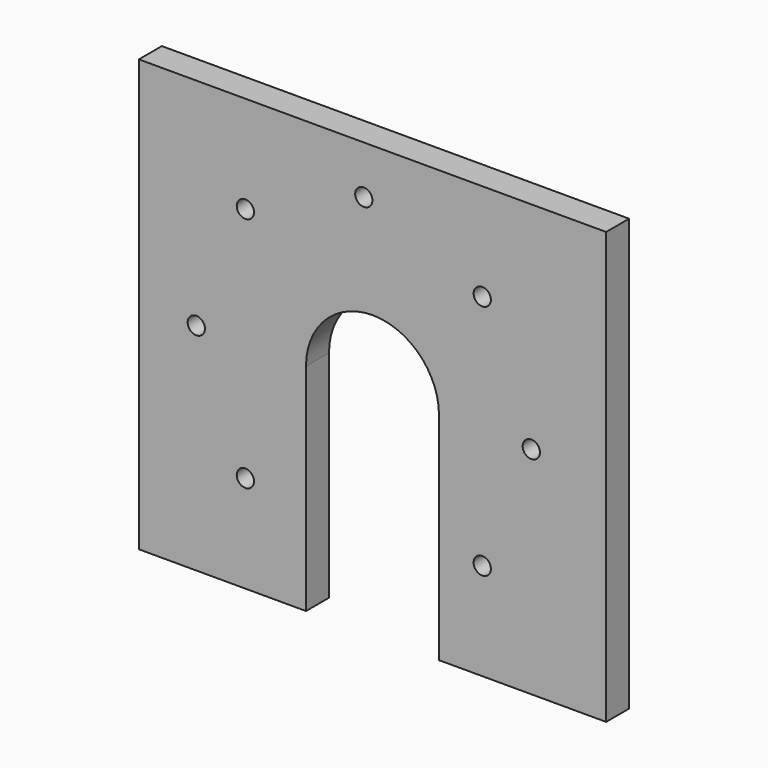
from build123d import *

# Parameters (mm, degrees)
F0_W             = 650
F0_H             = 600
F1_DEPTH         = 40
F3_DEPTH         = 40.001
F4_R             = 12
F5_DEPTH         = 40.001
F5_COPIES_COUNT  = 4
F5_COPIES_ANGLE  = 135
F5_COPIES1_COUNT = 4
F5_COPIES1_ANGLE = 135


# Not quite as in the source:
# - a pattern or mirror of a feature is missing from the dataset's text; its kind, count and spacing are read off the source's solid


with BuildPart() as f1:
    # F0 (on Front) → F1 (new body)
    with BuildSketch(Plane.XZ):
        with Locations((12.1025014669, -20.5410706814)):
            Rectangle(F0_W, F0_H)
    extrude(amount=F1_DEPTH)

    # F2 (on face) → F3 (cut, through all)
    with BuildSketch(Plane.XZ.offset(40)):
        with BuildLine():
            Line((-80.3974985331, -20.5410706814), (-80.3974985331, -320.5410706814))
            Line((-80.3974985331, -320.5410706814), (104.6025014669, -320.5410706814))
            Line((104.6025014669, -320.5410706814), (104.6025014669, -20.5410706814))
            ThreePointArc((104.6025014669, -20.5410706814), (12.1025014669, 71.9589293186), (-80.3974985331, -20.5410706814))
        make_face()
    extrude(amount=-F3_DEPTH, mode=Mode.SUBTRACT)

    # F4 (on face) → F5 (cut, through all)
    with BuildSketch(Plane.XZ.offset(40)):
        with Locations((0, 212.4589293186)):
            Circle(F4_R)
    f5 = extrude(amount=-F5_DEPTH, mode=Mode.SUBTRACT)

    # F5_copies: F5 ×4 about axis
    f5_copies_axis = Axis((0, 0, -20.541071), (0, 1, 0))
    for i in range(1, F5_COPIES_COUNT):
        add(f5.rotate(f5_copies_axis, i * F5_COPIES_ANGLE / (F5_COPIES_COUNT - 1)), mode=Mode.SUBTRACT)

    # F5_copies1: F5 ×4 about axis
    f5_copies1_axis = Axis((0, 0, -20.541071), (0, -1, 0))
    for i in range(1, F5_COPIES1_COUNT):
        add(f5.rotate(f5_copies1_axis, i * F5_COPIES1_ANGLE / (F5_COPIES1_COUNT - 1)), mode=Mode.SUBTRACT)


solid = f1.part
